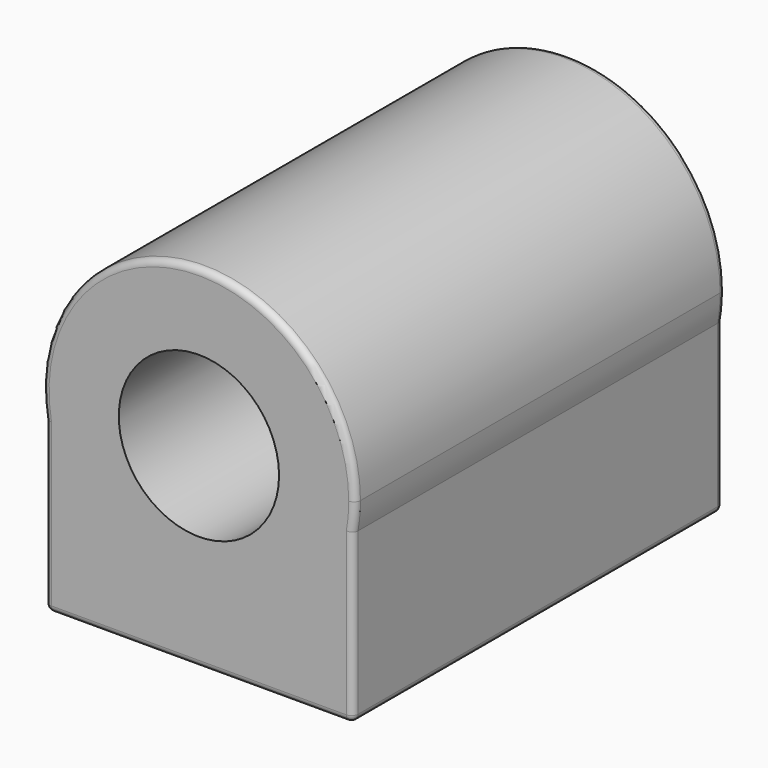
from build123d import *

# Parameters (mm, degrees)
F1_R     = 6.15
F2_DEPTH = 35.5
F3_DEPTH = 35.501
F4_DEPTH = 2
F5_R     = 0.5


# Not quite as in the source:
# - two fillets or chamfers of one size are made in one step


with BuildPart() as f2:
    # F1 (on face) → F2 (new body)
    with BuildSketch(Plane.XZ):
        Circle(F1_R)
    extrude(amount=F2_DEPTH)


with BuildPart() as f2b:
    # F0 (on Front) → F2, piece 2 (new body)
    with BuildSketch(Plane.XZ):
        with BuildLine():
            ThreePointArc((11.8124997243, -2.1130192291), (11.9530330187, -1.0606609515), (12, 0))
            ThreePointArc((12, 0), (-1.0606609515, 11.9530330187), (-11.8124997243, -2.1130192291))
            Line((-11.8124997243, -2.1130192291), (-11.8124997243, 1))
            Line((-11.8124997243, 1), (11.8124997243, 1))
            Line((11.8124997243, 1), (11.8124997243, -2.1130192291))
        make_face()
        with BuildLine():
            Line((-11.8124997243, 1), (-11.8124997243, -2.1130192291))
            ThreePointArc((-11.8124997243, -2.1130192291), (0, -12), (11.8124997243, -2.1130192291))
            Line((11.8124997243, -2.1130192291), (11.8124997243, 1))
            Line((11.8124997243, 1), (-11.8124997243, 1))
        make_face()
        with BuildLine():
            ThreePointArc((11.8124997243, -2.1130192291), (0, -12), (-11.8124997243, -2.1130192291))
            Line((-11.8124997243, -2.1130192291), (-11.8124997243, -13))
            Line((-11.8124997243, -13), (11.8124997243, -13))
            Line((11.8124997243, -13), (11.8124997243, -2.1130192291))
        make_face()
    extrude(amount=F2_DEPTH)


with BuildPart() as f3_tool:
    # F3 (cut, through all): a face of the model
    f3_faces = [f2.part.faces().sort_by_distance(p)[0] for p in [
        (0, -35.5, 0),
    ]]
    extrude(f3_faces, amount=-F3_DEPTH)


with BuildPart() as f2_1:
    add(f2.part)

    # F3: cut by f3_tool
    add(f3_tool.part, mode=Mode.SUBTRACT)


with BuildPart() as f2b_1:
    add(f2b.part)

    # F3: cut by f3_tool
    add(f3_tool.part, mode=Mode.SUBTRACT)

    # F4 (add): a face of the model
    f4_faces = [f2b_1.faces().sort_by_distance(p)[0] for p in [
        (0, -17.75, -13),
    ]]
    extrude(f4_faces, amount=F4_DEPTH)

    # F5
    f5_edges = [f2b_1.edges().sort_by_distance(p)[0] for p in [
        (0, -35.5, 12),
        (-11.8125, -35.5, -8.55651),
        (11.8125, -35.5, -8.55651),
        (11.8125, 0, -8.55651),
        (-11.8125, 0, -8.55651),
        (0, 0, 12),
        (-11.8125, -17.75, -15),
        (0, 0, -15),
        (11.8125, -17.75, -15),
        (0, -35.5, -15),
    ]]
    fillet(f5_edges, radius=F5_R)


solid = f2b_1.part
